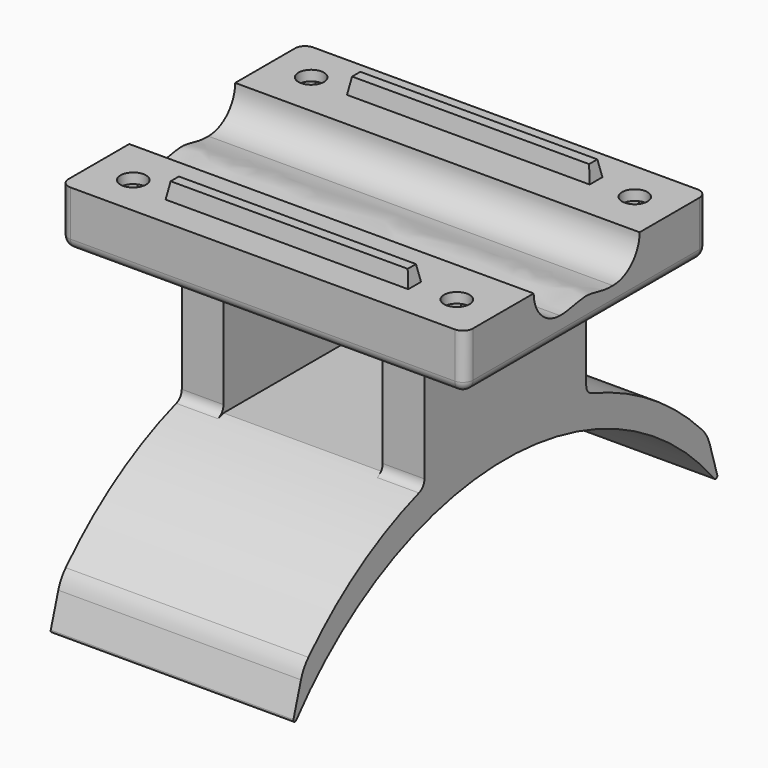
from build123d import *

# Parameters (mm, degrees)
F1_W          = 50.8
F1_H          = 38.1
F2_DEPTH      = 6.985
F4_DEPTH      = 50.8
F6_DEPTH      = 15.24
F6_DEPTH_BACK = 15.24
F7_W          = 20
F7_H          = 15.9418935353
F8_DEPTH      = 25.4
F9_R          = 1.6
F10_DEPTH     = 25.4
F11_R         = 1.6
F12_DEPTH     = 5.7
F13_W         = 30.48
F13_H         = 2
F14_DEPTH     = 2
F14_TAPER     = 10
F15_F1_R      = 0.254
F15_F2_R      = 0.254
F16_R         = 5.08
F17_R         = 1.27


# Not quite as in the source:
# - two fillets or chamfers of one size are made in one step


with BuildPart() as f2:
    # F1 (on Top) → F2 (new body)
    with BuildSketch(Plane.XY):
        Rectangle(F1_W, F1_H)
    extrude(amount=-F2_DEPTH)

    # F3 (on face) → F4 (cut, through all)
    with BuildSketch(Plane.YZ.offset(25.4)):
        with BuildLine():
            add(Edge.make_bspline(
                [(-4.125, 4.125), (-2.4255892558, 4.1137489608), (-0.0276085061, 2.971292738), (2.5249406681, 4.1137612248), (4.191, 4.191)],
                knots=[0, 0, 0, 0, 0.4977710734, 1, 1, 1, 1], degree=3))
            ThreePointArc((-4.125, 4.125), (-7.0418154724, 2.9168154724), (-8.25, 0))
            ThreePointArc((-8.25, 0), (-7.0418154724, -2.9168154724), (-4.125, -4.125))
            add(Edge.make_bspline(
                [(-4.125, -4.125), (-2.9335741419, -4.2006121948), (0.4172014685, -3.0581585459), (2.1438994445, -4.2006121948), (4.191, -4.191)],
                knots=[0, 0, 0, 0, 0.497799261, 1, 1, 1, 1], degree=3))
            ThreePointArc((4.191, -4.191), (7.15448452, -2.96348452), (8.382, 0))
            ThreePointArc((8.382, 0), (7.15448452, 2.96348452), (4.191, 4.191))
        make_face()
    extrude(amount=-F4_DEPTH, mode=Mode.SUBTRACT)

    # F5 (on Right) → F6 (join, two sides)
    with BuildSketch(Plane.YZ) as f6_sk:
        with BuildLine():
            ThreePointArc((-33.655, -41.5313687512), (0, -24.985), (33.655, -41.5313687512))
            Line((33.655, -41.5313687512), (31.75, -35.2327876972))
            ThreePointArc((31.75, -35.2327876972), (23.0609926669, -27.7856916423), (12.7, -22.9268935353))
            ThreePointArc((12.7, -22.9268935353), (0, -20.985), (-12.7, -22.9268935353))
            ThreePointArc((-12.7, -22.9268935353), (-23.0609926669, -27.7856916423), (-31.75, -35.2327876972))
            Line((-31.75, -35.2327876972), (-33.655, -41.5313687512))
        make_face()
        with BuildLine():
            ThreePointArc((-12.7, -22.9268935353), (0, -20.985), (12.7, -22.9268935353))
            Line((12.7, -22.9268935353), (12.7, -6.985))
            Line((12.7, -6.985), (-12.7, -6.985))
            Line((-12.7, -6.985), (-12.7, -22.9268935353))
        make_face()
    extrude(amount=F6_DEPTH)
    extrude(f6_sk.sketch, amount=-F6_DEPTH_BACK)

    # F7 (on face) → F8 (cut)
    with BuildSketch(Plane.XZ.offset(12.7)):
        with Locations((0, -14.9559467677)):
            Rectangle(F7_W, F7_H)
    extrude(amount=-F8_DEPTH, mode=Mode.SUBTRACT)

    # F9 (on face) → F10 (cut)
    with BuildSketch(Plane(origin=(0, 0, -6.985), x_dir=(1, 0, 0), z_dir=(0, 0, -1))):
        with Locations((20.32, -13.97)):
            Circle(F9_R)
        with Locations((-20.32, -13.97)):
            Circle(F9_R)
        with Locations((-20.32, 13.97)):
            Circle(F9_R)
        with Locations((20.32, 13.97)):
            Circle(F9_R)
    extrude(amount=-F10_DEPTH, mode=Mode.SUBTRACT)

    # F11 (on face) → F12 (cut)
    with BuildSketch(Plane(origin=(0, 0, -6.985), x_dir=(1, 0, 0), z_dir=(0, 0, -1))):
        Polygon((21.645, -16.26496732), (22.97, -13.97), (21.645, -11.67503268), (18.995, -11.67503268), (17.67, -13.97), (18.995, -16.26496732), align=None)
        with Locations((20.32, -13.97)):
            Circle(F11_R, mode=Mode.SUBTRACT)
        Polygon((-18.995, -11.67503268), (-21.645, -11.67503268), (-22.97, -13.97), (-21.645, -16.26496732), (-18.995, -16.26496732), (-17.67, -13.97), align=None)
        with Locations((-20.32, -13.97)):
            Circle(F11_R, mode=Mode.SUBTRACT)
        Polygon((-18.995, 11.67503268), (-17.67, 13.97), (-18.995, 16.26496732), (-21.645, 16.26496732), (-22.97, 13.97), (-21.645, 11.67503268), align=None)
        with Locations((-20.32, 13.97)):
            Circle(F11_R, mode=Mode.SUBTRACT)
        Polygon((18.995, 11.67503268), (21.645, 11.67503268), (22.97, 13.97), (21.645, 16.26496732), (18.995, 16.26496732), (17.67, 13.97), align=None)
        with Locations((20.32, 13.97)):
            Circle(F11_R, mode=Mode.SUBTRACT)
    extrude(amount=-F12_DEPTH, mode=Mode.SUBTRACT)

    # F13 (on face) → F14 (join)
    with BuildSketch(Plane.XY):
        with Locations((0, 14.24)):
            Rectangle(F13_W, F13_H)
        with Locations((0, -14.24)):
            Rectangle(F13_W, F13_H)
    extrude(amount=F14_DEPTH, taper=F14_TAPER)

    # F15: fillet of radius 0.254 on 2 edges, made by hand

    # F15_f1
    f15_f1_edges = [f2.edges().sort_by_distance(p)[0] for p in [
        (0, -33.655, -41.5313687512),
    ]]
    fillet(f15_f1_edges, radius=F15_F1_R)

    # F15_f2
    f15_f2_edges = [f2.edges().sort_by_distance(p)[0] for p in [
        (0, 33.655, -41.5313687512),
    ]]
    fillet(f15_f2_edges, radius=F15_F2_R)

    # F16
    f16_edges = [f2.edges().sort_by_distance(p)[0] for p in [
        (0, 31.75, -35.232788),
        (0, -31.75, -35.232788),
    ]]
    fillet(f16_edges, radius=F16_R)

    # F17
    f17_edges = [f2.edges().sort_by_distance(p)[0] for p in [
        (-15.24, 0, -6.985),
        (12.62, 12.7, -22.926894),
        (-12.62, 12.7, -22.926894),
        (-12.62, 12.7, -6.985),
        (0, 19.05, -6.985),
        (25.4, 0, -6.985),
        (-25.4, 0, -6.985),
        (0, -19.05, -6.985),
        (-12.62, -12.7, -6.985),
        (-10, 0, -6.985),
        (12.62, -12.7, -6.985),
        (15.24, 0, -6.985),
        (10, 0, -6.985),
        (12.62, 12.7, -6.985),
        (-12.62, -12.7, -22.926894),
        (12.62, -12.7, -22.926894),
        (25.4, 19.05, -3.4925),
        (-25.4, 19.05, -3.4925),
        (25.4, -19.05, -3.4925),
        (-25.4, -19.05, -3.4925),
    ]]
    fillet(f17_edges, radius=F17_R)


solid = f2.part
